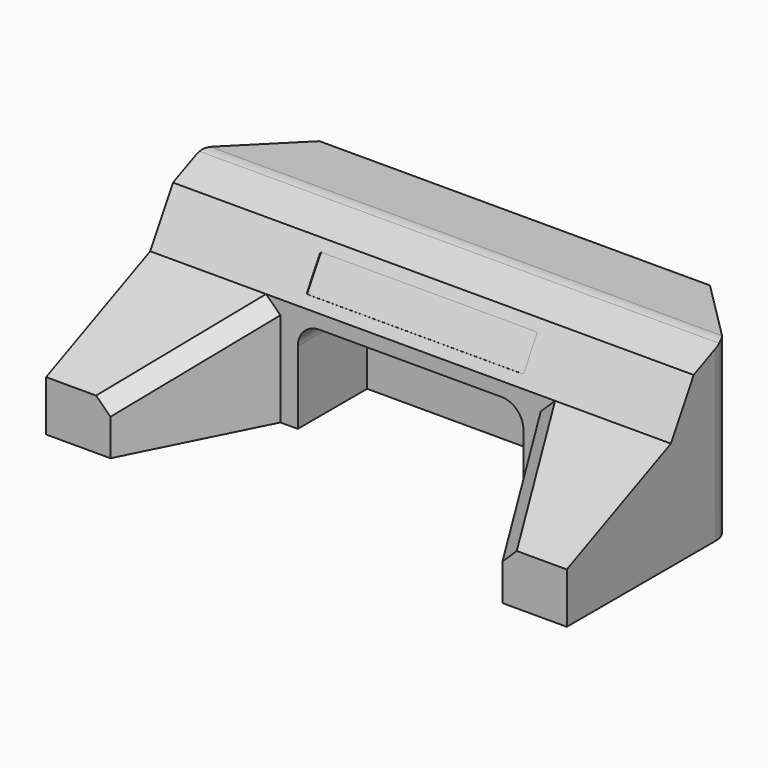
from build123d import *

# Parameters (mm, degrees)
F1_DEPTH = 2000
F3_DEPTH = 6000.001
F4_SIZE  = 150
F5_W     = 2600
F5_H     = 1087.6065318632
F6_DEPTH = 1000
F7_W     = 2500
F7_H     = 400
F8_DEPTH = 10
F9_R     = 19.313708499
F10_F1_R = 242.7414236909
F10_F2_R = 242.7414236909
F10_F3_R = 242.7414236909
F11_R    = 250


with BuildPart() as f1:
    # F0 (on Top) → F1 (new body)
    with BuildSketch(Plane.XY):
        Polygon((-3000, -1500), (-2258.4035396576, -1500), (-1500, 0), (1500, 0), (2258.4035396576, -1500), (3000, -1500), (3000, 750), (2250, 1500), (-2250, 1500), (-3000, 750), align=None)
    extrude(amount=F1_DEPTH)

    # F2 (on face) → F3 (cut, through all)
    with BuildSketch(Plane(origin=(-3000, 0, 0), x_dir=(0, -1, 0), z_dir=(-1, 0, 0))):
        Polygon((1500, 2000), (-750, 2000), (-327.833239258, 1812.3703285591), (1500, 1000), align=None)
        Polygon((1500, 1000), (-327.833239258, 1812.3703285591), (0, 1248.974442482), (1500, 582.3077758153), align=None)
    extrude(amount=-F3_DEPTH, mode=Mode.SUBTRACT)

    # F4
    f4_edges = [f1.edges().sort_by_distance(p)[0] for p in [
        (-1879.20177, -750, 915.641109),
        (1879.20177, -750, 915.641109),
    ]]
    chamfer(f4_edges, length=F4_SIZE)

    # F5 (on face) → F6 (cut)
    with BuildSketch(Plane.XZ):
        with Locations((0, 543.8032659316)):
            Rectangle(F5_W, F5_H)
    extrude(amount=-F6_DEPTH, mode=Mode.SUBTRACT)

    # F7 (on face) → F8 (cut)
    with BuildSketch(Plane(origin=(0, -542.9303888793, 315.9246144256), x_dir=(1, 0, 0), z_dir=(0, -0.86432215, 0.5029385858))):
        with Locations((0, 1405.4340400094)):
            Rectangle(F7_W, F7_H)
    extrude(amount=-F8_DEPTH, mode=Mode.SUBTRACT)

    # F9
    f9_edges = [f1.edges().sort_by_distance(p)[0] for p in [
        (-1250, 67.650513, 1355.293263),
        (-1250, 268.825948, 1701.022123),
        (1250, 268.825948, 1701.022123),
        (1250, 67.650513, 1355.293263),
    ]]
    fillet(f9_edges, radius=F9_R)

    # F10: fillet of radius 242.7414236909 on 3 edges, made by hand

    # F10_f1
    f10_f1_edges = [f1.edges().sort_by_distance(p)[0] for p in [
        (-3000, 750, 1000),
    ]]
    fillet(f10_f1_edges, radius=F10_F1_R)

    # F10_f2
    f10_f2_edges = [f1.edges().sort_by_distance(p)[0] for p in [
        (10.9015511853, 750, 2000),
    ]]
    fillet(f10_f2_edges, radius=F10_F2_R)

    # F10_f3
    f10_f3_edges = [f1.edges().sort_by_distance(p)[0] for p in [
        (3000, 750, 997.2355539079),
    ]]
    fillet(f10_f3_edges, radius=F10_F3_R)

    # F11
    f11_edges = [f1.edges().sort_by_distance(p)[0] for p in [
        (-1300, 500, 1087.606532),
        (1300, 500, 1087.606532),
    ]]
    fillet(f11_edges, radius=F11_R)


solid = f1.part
